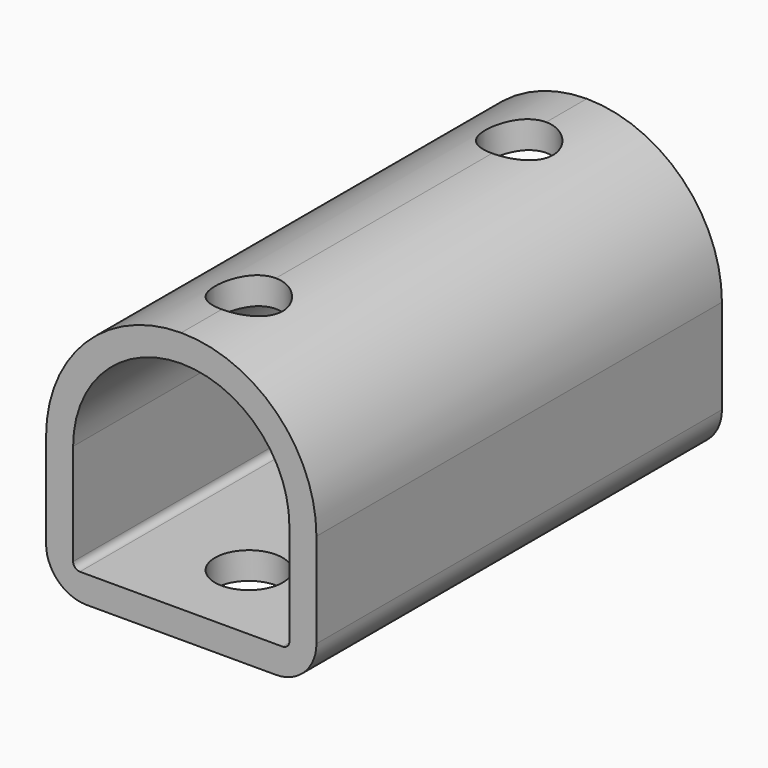
from build123d import *

# Parameters (mm, degrees)
F0_W        = 40
F0_H        = 75
F1_DEPTH    = 40
F3_D        = 10
F4_T1_DEPTH = 175
F5_T1_DEPTH = 175
F6_R        = 6
F8_DEPTH    = 75.0010001
F9_R        = 1


# Not quite as in the source:
# - a fillet or chamfer that OpenCascade refuses, or shapes differently, is made with other operations: its cross-section is extruded or revolved along the edge and cut away or added


with BuildPart() as f1:
    # F0 (on Top) → F1 (new body)
    with BuildSketch(Plane.XY):
        Rectangle(F0_W, F0_H)
    extrude(amount=F1_DEPTH)

    # F3 (through all)
    with Locations(Plane.XY.offset(40)):
        with Locations((0, 25), (0, -25)):
            Hole(F3_D / 2)

    # F4: fillet of radius 20 on 1 edges, made by hand

    # F4_s2 → F4_t1 (cut)
    with BuildSketch(Plane.XZ.offset(-87.5)):
        with BuildLine():
            ThreePointArc((20, 20), (14.1421356237, 34.1421356237), (0, 40))
            Line((0, 40), (20, 40))
            Line((20, 40), (20, 20))
        make_face()
    extrude(amount=F4_T1_DEPTH, mode=Mode.SUBTRACT)

    # F5: fillet of radius 20 on 1 edges, made by hand

    # F5_s2 → F5_t1 (cut)
    with BuildSketch(Plane.XZ.offset(-87.5)):
        with BuildLine():
            ThreePointArc((-20, 20), (-14.1421356237, 34.1421356237), (0, 40))
            Line((0, 40), (-20, 40))
            Line((-20, 40), (-20, 20))
        make_face()
    extrude(amount=F5_T1_DEPTH, mode=Mode.SUBTRACT)

    # F6
    f6_edges = [f1.edges().sort_by_distance(p)[0] for p in [
        (-20, 0, 0),
        (20, 0, 0),
    ]]
    fillet(f6_edges, radius=F6_R)

    # F7 (on face) → F8 (cut, through all)
    with BuildSketch(Plane.XZ.offset(37.5)):
        with BuildLine():
            Line((-16, 20), (-16, 4))
            Line((-16, 4), (16, 4))
            Line((16, 4), (16, 20))
            ThreePointArc((16, 20), (0, 36), (-16, 20))
        make_face()
    extrude(amount=-F8_DEPTH, mode=Mode.SUBTRACT)

    # F9
    f9_edges = [f1.edges().sort_by_distance(p)[0] for p in [
        (-16, 0, 4),
        (16, 0, 4),
    ]]
    fillet(f9_edges, radius=F9_R)


solid = f1.part
